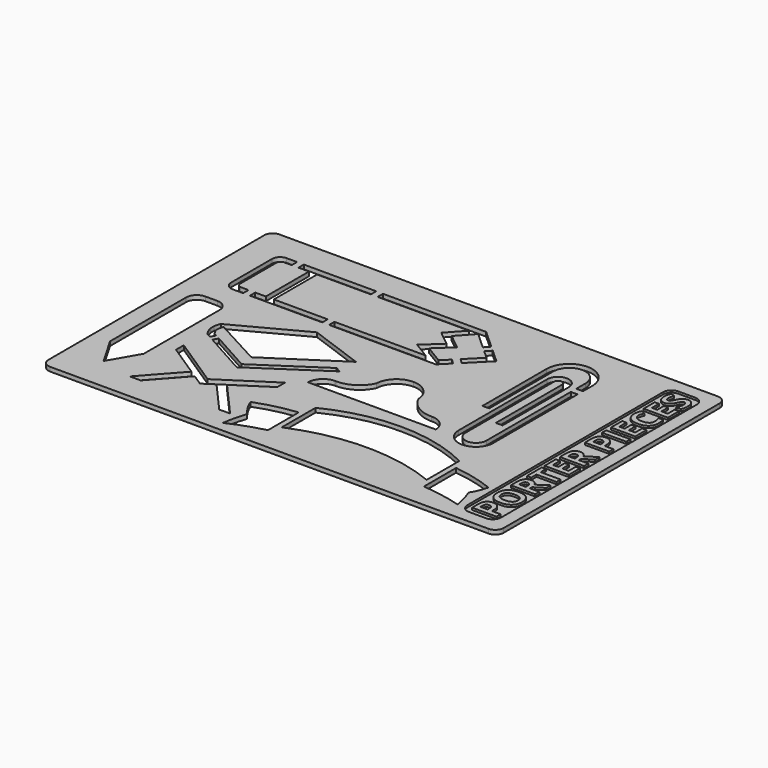
from build123d import *

# Parameters (mm, degrees)
F0_W         = 85.725
F0_H         = 53.975
F1_DEPTH     = 0.79375
F2_R         = 1.5875
F3_W         = 6.35
F3_H         = 49.2125
F4_DEPTH     = 0.396875
F5_R         = 1.5875
F6_TEXT_SIZE = 6.4051106395
F7_DEPTH     = 0.396875
F9_DEPTH     = 25.4
F11_DEPTH    = 25.4
F13_DEPTH    = 25.4
F15_DEPTH    = 25.4
F17_DEPTH    = 25.4
F19_DEPTH    = 25.4
F21_DEPTH    = 25.4
F23_DEPTH    = 25.4
F25_DEPTH    = 25.4


# Not quite as in the source:
# - Text() gives the source's letters only with a copy of the font that has no kerning and outlines rounded to 1/6400 em; it was checked with that copy


with BuildPart() as f1:
    # F0 (on Top) → F1 (new body)
    with BuildSketch(Plane.XY):
        Rectangle(F0_W, F0_H)
    extrude(amount=F1_DEPTH)

    # F2
    f2_edges = [f1.edges().sort_by_distance(p)[0] for p in [
        (42.8625, 26.9875, 0.396875),
        (-42.8625, 26.9875, 0.396875),
        (-42.8625, -26.9875, 0.396875),
        (42.8625, -26.9875, 0.396875),
    ]]
    fillet(f2_edges, radius=F2_R)

    # F3 (on face) → F4 (cut)
    with BuildSketch(Plane.XY.offset(0.79375)):
        with Locations((37.30625, 0)):
            Rectangle(F3_W, F3_H)
    extrude(amount=-F4_DEPTH, mode=Mode.SUBTRACT)

    # F5
    f5_edges = [f1.edges().sort_by_distance(p)[0] for p in [
        (34.13125, -24.60625, 0.595313),
        (40.48125, -24.60625, 0.595313),
        (40.48125, 24.60625, 0.595313),
        (34.13125, 24.60625, 0.595313),
    ]]
    fillet(f5_edges, radius=F5_R)

    # F6 (on face) → F7 (join)
    with BuildSketch(Plane.XY.offset(0.396875)):
        with Locations(Location((39.7566241945, -23.8125), (0, 0, 90))):
            Text('PORTER PIECES', F6_TEXT_SIZE, font='Open Sans', font_style=FontStyle.BOLD, text_align=(TextAlign.LEFT, TextAlign.BOTTOM))
    extrude(amount=F7_DEPTH)

    # F8 (on face) → F9 (cut)
    with BuildSketch(Plane.XY.offset(0.79375)):
        with BuildLine():
            Line((-33.7677486241, 21.7466053596), (-35.7372550855, 21.7466053596))
            ThreePointArc((-35.7372550855, 21.7466053596), (-36.81488582, 21.3002360941), (-37.2612550855, 20.2226053596))
            Line((-37.2612550855, 20.2226053596), (-37.2612550855, 10.5706053596))
            ThreePointArc((-37.2612550855, 10.5706053596), (-36.81488582, 9.492974625), (-35.7372550855, 9.0466053596))
            Line((-35.7372550855, 9.0466053596), (-33.7677486241, 9.0466053596))
            Line((-33.7677486241, 9.0466053596), (-33.7677486241, 10.3166053596))
            Line((-33.7677486241, 10.3166053596), (-35.2292550855, 10.3166053596))
            ThreePointArc((-35.2292550855, 10.3166053596), (-35.7680704527, 10.5397899923), (-35.9912550855, 11.0786053596))
            Line((-35.9912550855, 11.0786053596), (-35.9912550855, 19.7146053596))
            ThreePointArc((-35.9912550855, 19.7146053596), (-35.7680704527, 20.2534207268), (-35.2292550855, 20.4766053596))
            Line((-35.2292550855, 20.4766053596), (-33.7677486241, 20.4766053596))
            Line((-33.7677486241, 20.4766053596), (-33.7677486241, 21.7466053596))
        make_face()
        Polygon((5.3826721636, 18.5391742673), (1.8361794882, 21.7466053596), (-17.5816844064, 21.7466053596), (-17.5816844064, 20.4766053596), (-0.3652806475, 20.4766053596), (-3.1391682707, 17.4094865797), (-0.363157008, 15.1634403795), (-3.5310297481, 12.2083263772), (-0.4232278817, 10.3166053596), (-17.5816844064, 10.3166053596), (-17.5816844064, 9.0466053596), (2.5477347284, 9.0466053596), (4.3244664298, 10.8346818394), (3.4235874695, 11.7298450083), (2.0193143784, 10.3166053596), (-1.4398970319, 12.4222295951), (1.5717184313, 15.2315807765), (-1.2972053613, 17.5528016844), (1.3470687635, 20.4766053596), (4.5308021701, 17.5972520231), align=None)
        Polygon((5.2197851689, 11.7357173633), (8.8574459912, 15.3966053596), (6.3264284596, 17.685645566), (5.4745584661, 16.7437233218), (7.0183315829, 15.3475422641), (4.3189062086, 12.6308805322), align=None)
        Polygon((-32.4977486241, 20.4766053596), (-30.5072068027, 20.4766053596), (-30.5072068027, 10.3166053596), (-32.4977486241, 10.3166053596), (-32.4977486241, 9.0466053596), (-18.8516844064, 9.0466053596), (-18.8516844064, 10.3166053596), (-28.9892590395, 10.3166053596), (-28.9892590395, 20.4766053596), (-18.8516844064, 20.4766053596), (-18.8516844064, 21.7466053596), (-32.4977486241, 21.7466053596), align=None)
    extrude(amount=-F9_DEPTH, mode=Mode.SUBTRACT)

    # F10 (on face) → F11 (cut)
    with BuildSketch(Plane.XY.offset(0.79375)):
        with BuildLine():
            Line((16.1392502487, 3.001535777), (17.4092501402, 3.001535777))
            Line((17.4092501402, 3.001535777), (17.4092501402, 18.0616676807))
            ThreePointArc((17.4092501402, 18.0616676807), (20.4522218555, 21.1046393961), (23.4951935709, 18.0616676807))
            Line((23.4951935709, 18.0616676807), (23.4951935709, 15.8782023937))
            Line((23.4951935709, 15.8782023937), (24.7651934624, 15.8782023937))
            Line((24.7651934624, 15.8782023937), (24.7651934624, 18.0616676807))
            ThreePointArc((24.7651934624, 18.0616676807), (20.4522218555, 22.3746392876), (16.1392502487, 18.0616676807))
            Line((16.1392502487, 18.0616676807), (16.1392502487, 3.001535777))
        make_face()
        with BuildLine():
            ThreePointArc((23.4951935709, -5.2505913191), (21.514586173, -7.2311987169), (19.5339787751, -5.2505913191))
            Line((19.5339787751, -5.2505913191), (19.5339787751, 15.5860306695))
            ThreePointArc((19.5339787751, 15.5860306695), (20.2959787751, 16.3480306695), (21.0579787751, 15.5860306695))
            Line((21.0579787751, 15.5860306695), (21.0579787751, 0))
            Line((21.0579787751, 0), (22.3279786667, 0))
            Line((22.3279786667, 0), (22.3279786667, 15.5860306695))
            ThreePointArc((22.3279786667, 15.5860306695), (20.2959787751, 17.618030561), (18.2639788836, 15.5860306695))
            Line((18.2639788836, 15.5860306695), (18.2639788836, -5.2505913191))
            ThreePointArc((18.2639788836, -5.2505913191), (21.514586173, -8.5011986084), (24.7651934624, -5.2505913191))
            Line((24.7651934624, -5.2505913191), (24.7651934624, 14.6082023937))
            Line((24.7651934624, 14.6082023937), (23.4951935709, 14.6082023937))
            Line((23.4951935709, 14.6082023937), (23.4951935709, -5.2505913191))
        make_face()
    extrude(amount=-F11_DEPTH, mode=Mode.SUBTRACT)

    # F12 (on face) → F13 (cut)
    with BuildSketch(Plane.XY.offset(0.79375)):
        with BuildLine():
            Line((-35.1528163023, 4.7625), (-37.4388163023, 4.7625))
            ThreePointArc((-37.4388163023, 4.7625), (-38.8756572817, 4.1673409794), (-39.4708163023, 2.7305))
            Line((-39.4708163023, 2.7305), (-39.4708163023, -15.138238686))
            Line((-39.4708163023, -15.138238686), (-36.2958163023, -20.6375))
            Line((-36.2958163023, -20.6375), (-33.1208163023, -15.138238686))
            Line((-33.1208163023, -15.138238686), (-33.1208163023, 2.7305))
            ThreePointArc((-33.1208163023, 2.7305), (-33.7159753229, 4.1673409794), (-35.1528163023, 4.7625))
        make_face()
    extrude(amount=-F13_DEPTH, mode=Mode.SUBTRACT)

    # F14 (on face) → F15 (cut)
    with BuildSketch(Plane.XY.offset(0.79375)):
        with BuildLine():
            Line((-17.5054054707, 6.0904221609), (-30.1968231797, -0.6564526702))
            ThreePointArc((-30.1968231797, -0.6564526702), (-30.4228781029, -1.2417662409), (-30.5364560529, -1.8588503953))
            ThreePointArc((-30.5364560529, -1.8588503953), (-30.5567634681, -2.2573976299), (-30.5128966782, -2.6540435602))
            ThreePointArc((-30.5128966782, -2.6540435602), (-30.2170789188, -3.6169279755), (-29.6497810632, -4.4492906891))
            Line((-29.6497810632, -4.4492906891), (-28.9375586401, -4.8461378753))
            Line((-28.9375586401, -4.8461378753), (-28.416797737, -3.9441535327))
            Line((-28.416797737, -3.9441535327), (-28.9851379085, -3.6274769012))
            ThreePointArc((-28.9851379085, -3.6274769012), (-29.202628888, -3.3103059399), (-29.3649111678, -2.9616453507))
            ThreePointArc((-29.3649111678, -2.9616453507), (-29.5107198712, -2.560854109), (-29.5081973729, -2.1343714782))
            ThreePointArc((-29.5081973729, -2.1343714782), (-29.4480123861, -1.6310876817), (-29.2802819432, -1.1527746973))
            Line((-29.2802819432, -1.1527746973), (-20.0947467238, -6.1268918216))
            Line((-20.0947467238, -6.1268918216), (-7.1480404586, 2.3340540938))
            Line((-7.1480404586, 2.3340540938), (-17.5054054707, 6.0904221609))
        make_face()
        Polygon((-28.0500334717, -5.3406629764), (-19.7665207088, -9.9561996758), (-7.1115707979, -1.5317230718), (-8.1501237438, -0.9720407724), (-19.8146875051, -8.7372113337), (-27.5292725687, -4.4386786337), align=None)
    extrude(amount=-F15_DEPTH, mode=Mode.SUBTRACT)

    # F16 (on face) → F17 (cut)
    with BuildSketch(Plane.XY.offset(0.79375)):
        with BuildLine():
            ThreePointArc((7.3943778518, -1.1470840846), (6.173140208, 1.5384868862), (3.4348527927, 2.6364371827))
            ThreePointArc((3.4348527927, 2.6364371827), (0.6965653775, 1.5384868862), (-0.5246722663, -1.1470840846))
            ThreePointArc((-0.5246722663, -1.1470840846), (-2.5653688403, -3.4674104806), (-5.5335197843, -4.3267340892))
            ThreePointArc((-5.5335197843, -4.3267340892), (-5.6507179766, -4.3252547265), (-5.7678583032, -4.3212862672))
            ThreePointArc((-5.7678583032, -4.3212862672), (-7.750310457, -5.1635440927), (-8.5904113948, -7.1469112299))
            Line((-8.5904113948, -7.1469112299), (3.4348527927, -7.1469112299))
            Line((3.4348527927, -7.1469112299), (15.4601169803, -7.1469112299))
            ThreePointArc((15.4601169803, -7.1469112299), (14.6200160425, -5.1635440927), (12.6375638886, -4.3212862672))
            ThreePointArc((12.6375638886, -4.3212862672), (12.520423562, -4.3252547265), (12.4032253697, -4.3267340892))
            ThreePointArc((12.4032253697, -4.3267340892), (9.4350744257, -3.4674104806), (7.3943778518, -1.1470840846))
        make_face()
        with BuildLine():
            ThreePointArc((-5.7678583032, -4.3212862672), (-5.6507179766, -4.3252547265), (-5.5335197843, -4.3267340892))
            ThreePointArc((-5.5335197843, -4.3267340892), (-5.6506334686, -4.3216196083), (-5.7678583032, -4.3212862672))
        make_face()
        with BuildLine():
            ThreePointArc((12.6375638886, -4.3212862672), (12.520339054, -4.3216196083), (12.4032253697, -4.3267340892))
            ThreePointArc((12.4032253697, -4.3267340892), (12.520423562, -4.3252547265), (12.6375638886, -4.3212862672))
        make_face()
    extrude(amount=-F17_DEPTH, mode=Mode.SUBTRACT)

    # F18 (on face) → F19 (cut)
    with BuildSketch(Plane.XY.offset(0.79375)):
        Polygon((-20.7396529175, -15.5789796263), (-30.2149746567, -9.3559667796), (-30.2149746567, -11.17925585), (-24.0908778497, -15.2013180189), (-30.2149746567, -22.0559667796), (-28.1636461176, -22.0559667796), (-22.7981031571, -16.0503607998), (-20.744000428, -17.3994134255), (-18.6834776246, -16.0601872366), (-13.3466805534, -22.0913522539), (-11.3329460338, -22.0586911371), (-11.3353567361, -22.0559667796), (-17.3866623797, -15.217328844), (-11.1649746567, -11.1735749367), (-11.1649746567, -9.3559667796), align=None)
        Polygon((-11.1649746567, -22.0559667796), (-11.3353567361, -22.0559667796), (-11.3329460338, -22.0586911371), align=None)
    extrude(amount=-F19_DEPTH, mode=Mode.SUBTRACT)

    # F20 (on face) → F21 (cut)
    with BuildSketch(Plane.XY.offset(0.79375)):
        with BuildLine():
            Line((-2.64955475, -12.8012718633), (-2.64955475, -20.7663550973))
            ThreePointArc((-2.64955475, -20.7663550973), (10.8646334433, -17.9353931629), (24.4317278266, -20.5008517951))
            Line((24.4317278266, -20.5008517951), (24.4317278266, -12.8012718633))
            ThreePointArc((24.4317278266, -12.8012718633), (10.8910865383, -9.6149485633), (-2.64955475, -12.8012718633))
        make_face()
    extrude(amount=-F21_DEPTH, mode=Mode.SUBTRACT)

    # F22 (on face) → F23 (cut)
    with BuildSketch(Plane.XY.offset(0.79375)):
        with BuildLine():
            Line((-3.66555475, -22.7326467496), (-3.66555475, -15.490947109))
            ThreePointArc((-3.66555475, -15.490947109), (-7.5349471108, -16.1555552429), (-11.28555475, -17.3160911322))
            ThreePointArc((-11.28555475, -17.3160911322), (-10.4189526543, -19.0775277598), (-9.2351608393, -20.6435083229))
            ThreePointArc((-9.2351608393, -20.6435083229), (-9.8781005618, -22.8284225891), (-10.286215779, -25.0691063702))
            ThreePointArc((-10.286215779, -25.0691063702), (-7.0341071439, -23.7358973217), (-3.66555475, -22.7326467496))
        make_face()
    extrude(amount=-F23_DEPTH, mode=Mode.SUBTRACT)

    # F24 (on face) → F25 (cut)
    with BuildSketch(Plane.XY.offset(0.79375)):
        with BuildLine():
            ThreePointArc((33.0677278266, -16.7272731821), (29.3164193394, -15.5444680941), (25.4477278266, -14.8341377333))
            Line((25.4477278266, -14.8341377333), (25.4477278266, -22.4221740468))
            ThreePointArc((25.4477278266, -22.4221740468), (29.2085218738, -22.9119819627), (32.8997092513, -23.7829695656))
            ThreePointArc((32.8997092513, -23.7829695656), (32.433628128, -21.7729481723), (31.783208251, -19.8147930205))
            ThreePointArc((31.783208251, -19.8147930205), (32.5448564417, -18.3207029815), (33.0677278266, -16.7272731821))
        make_face()
    extrude(amount=-F25_DEPTH, mode=Mode.SUBTRACT)


solid = f1.part
